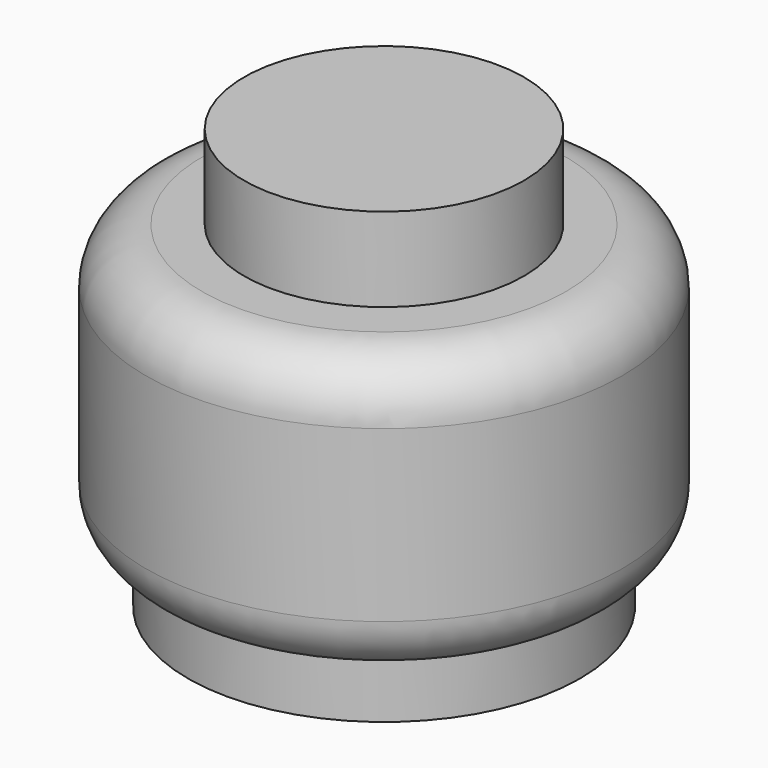
from build123d import *

# Parameters (mm, degrees)
F0_R     = 3.5
F1_DEPTH = 1
F2_R     = 4.25
F3_DEPTH = 5
F4_R     = 2.5
F5_DEPTH = 1.5
F7_R     = 2.5
F8_DEPTH = 6


# Not quite as in the source:
# - a fillet or chamfer that OpenCascade refuses, or shapes differently, is made with other operations: its cross-section is extruded or revolved along the edge and cut away or added


with BuildPart() as f1:
    # F0 (on Top) → F1 (new body)
    with BuildSketch(Plane.XY):
        Circle(F0_R)
    extrude(amount=F1_DEPTH)

    # F2 (on face) → F3 (join)
    with BuildSketch(Plane.XY.offset(1)):
        Circle(F2_R)
    extrude(amount=F3_DEPTH)

    # F6: fillet of radius 1 on 2 edges, made by hand

    # F6_s1 → F6_t2 (revolve, cut)
    with BuildSketch(Plane.XZ):
        with BuildLine():
            ThreePointArc((4.25, 5), (3.9571067812, 5.7071067812), (3.25, 6))
            Line((3.25, 6), (4.25, 6))
            Line((4.25, 6), (4.25, 5))
        make_face()
    revolve(axis=Axis((0, 0, 6), (0, 0, 1)), mode=Mode.SUBTRACT)

    # F6_s3 → F6_t4 (revolve, cut)
    with BuildSketch(Plane.XZ):
        with BuildLine():
            ThreePointArc((4.25, 1.9682458366), (4.040569415, 1.3558734009), (3.5, 1))
            Line((3.5, 1), (4.25, 1))
            Line((4.25, 1), (4.25, 1.9682458366))
        make_face()
    revolve(axis=Axis((0, 0, 1), (0, 0, 1)), mode=Mode.SUBTRACT)

    # F7 (on face) → F8 (cut)
    with BuildSketch(Plane(origin=(0, 0, 0), x_dir=(1, 0, 0), z_dir=(0, 0, -1))):
        Circle(F7_R)
    extrude(amount=-F8_DEPTH, mode=Mode.SUBTRACT)


with BuildPart() as f5:
    # F4 (on face) → F5 (new body)
    with BuildSketch(Plane.XY.offset(6)):
        Circle(F4_R)
    extrude(amount=F5_DEPTH)


solid = Compound([f1.part, f5.part])
